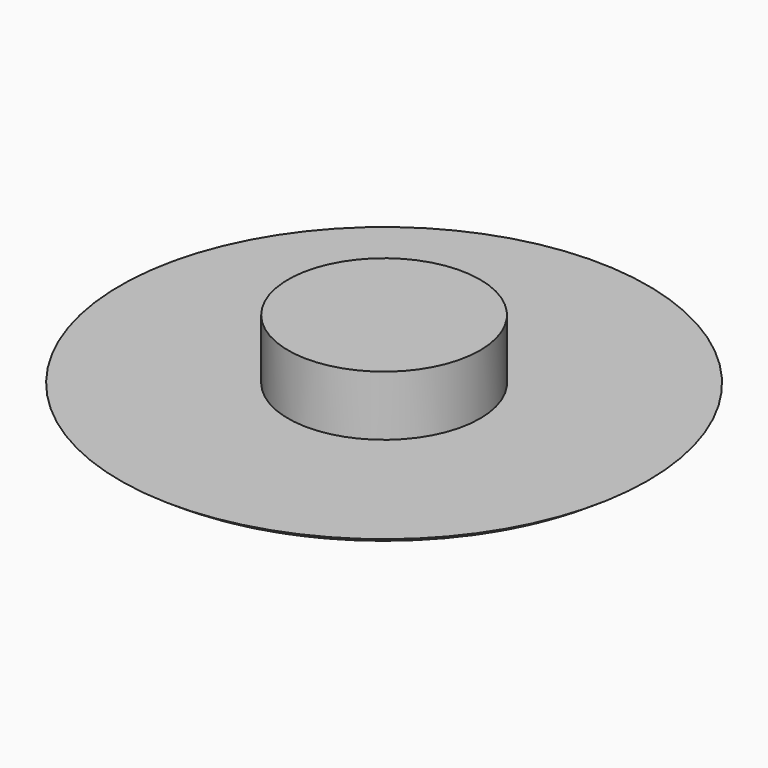
from build123d import *

# Parameters (mm, degrees)
F0_R     = 4
F1_DEPTH = 3.5
F0_R_2   = 11
F2_DEPTH = 1
F4_DEPTH = 0.5


# Not quite as in the source:
# - a fillet or chamfer that OpenCascade refuses, or shapes differently, is made with other operations: its cross-section is extruded or revolved along the edge and cut away or added


with BuildPart() as f1:
    # F0 (on Top) → F1 (new body)
    with BuildSketch(Plane.XY):
        Circle(F0_R)
    extrude(amount=F1_DEPTH)

    # F0 (on Top) → F2 (join)
    with BuildSketch(Plane.XY):
        Circle(F0_R_2)
        Circle(F0_R, mode=Mode.SUBTRACT)
    extrude(amount=F2_DEPTH)

    # F3 (on face) → F4 (cut)
    with BuildSketch(Plane.XY):
        with BuildLine():
            Line((-0.6011938094, -3.9545626817), (-0.6011938094, -7.9646864906))
            ThreePointArc((-0.6011938094, -7.9646864906), (0, -8.523200555), (0.6011938094, -7.9646864906))
            Line((0.6011938094, -7.9646864906), (0.6011938094, -3.9545626817))
            ThreePointArc((0.6011938094, -3.9545626817), (0, -4), (-0.6011938094, -3.9545626817))
        make_face()
        with BuildLine():
            Line((-0.6011938094, 0), (-0.6011938094, -3.9545626817))
            ThreePointArc((-0.6011938094, -3.9545626817), (0, -4), (0.6011938094, -3.9545626817))
            Line((0.6011938094, -3.9545626817), (0.6011938094, 0))
            ThreePointArc((0.6011938094, 0), (0, 0.6491973737), (-0.6011938094, 0))
        make_face()
        with BuildLine():
            ThreePointArc((-1.7606344773, -6.5513337031), (0, 6.8746740692), (1.7606344773, -6.5513337031))
            ThreePointArc((1.7606344773, -6.5513337031), (1.5154543616, -7.2599851451), (2.1851049368, -7.5974288625))
            ThreePointArc((2.1851049368, -7.5974288625), (2.2008228493, -7.5929180655), (2.21653145, -7.5883749472))
            ThreePointArc((2.21653145, -7.5883749472), (0, 7.9960832706), (-2.21653145, -7.5883749472))
            ThreePointArc((-2.21653145, -7.5883749472), (-2.2008228493, -7.5929180655), (-2.1851049368, -7.5974288625))
            ThreePointArc((-2.1851049368, -7.5974288625), (-1.5154543616, -7.2599851451), (-1.7606344773, -6.5513337031))
        make_face()
    extrude(amount=F4_DEPTH, mode=Mode.SUBTRACT)

    # F5: fillet of radius 5.08 on 1 edges, made by hand

    # F5_s1 → F5_t2 (revolve, cut)
    with BuildSketch(Plane.XZ):
        with BuildLine():
            ThreePointArc((11, 1), (9.567188555, 0.2564743185), (7.9734508099, 0))
            Line((7.9734508099, 0), (11, 0))
            Line((11, 0), (11, 1))
        make_face()
    revolve(axis=Axis((0, 0, 0), (0, 0, 1)), mode=Mode.SUBTRACT)


solid = f1.part
